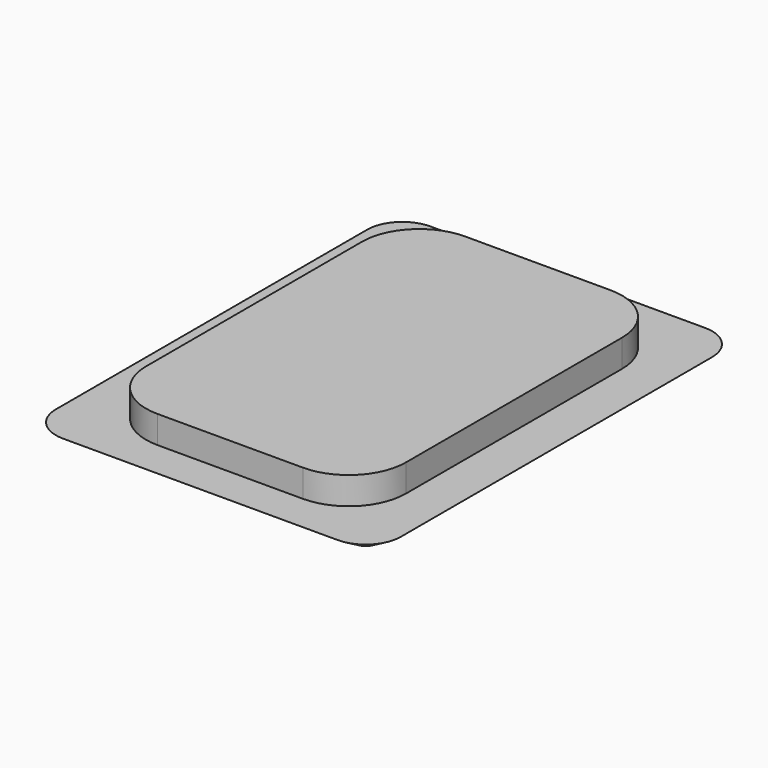
from build123d import *

# Parameters (mm, degrees)
F2_DEPTH     = 1.524
F3_DEPTH     = 0.762
F4_T1_DEPTH  = 21.59
F4_T3_DEPTH  = 15.24
F4_T6_ANGLE  = 90
F4_T8_ANGLE  = 90
F4_T10_ANGLE = 90
F4_T12_ANGLE = 90


# Not quite as in the source:
# - a fillet or chamfer that OpenCascade refuses, or shapes differently, is made with other operations: its cross-section is extruded or revolved along the edge and cut away or added


with BuildPart() as f2:
    # F1 (on face) → F2 (new body)
    with BuildSketch(Plane.XY):
        with BuildLine():
            ThreePointArc((-45.0744511747, 18.5649100114), (-44.144515205, 16.3198459811), (-41.8994511747, 15.3899100114))
            Line((-41.8994511747, 15.3899100114), (-33.8222511747, 15.3899100114))
            ThreePointArc((-33.8222511747, 15.3899100114), (-31.5771871445, 16.3198459811), (-30.6472511747, 18.5649100114))
            Line((-30.6472511747, 18.5649100114), (-30.6472511747, 33.5509100114))
            ThreePointArc((-30.6472511747, 33.5509100114), (-31.5771871445, 35.7959740417), (-33.8222511747, 36.7259100114))
            Line((-33.8222511747, 36.7259100114), (-41.8994511747, 36.7259100114))
            ThreePointArc((-41.8994511747, 36.7259100114), (-44.144515205, 35.7959740417), (-45.0744511747, 33.5509100114))
            Line((-45.0744511747, 33.5509100114), (-45.0744511747, 18.5649100114))
        make_face()
    extrude(amount=F2_DEPTH)

    # F0 (on Top) → F3 (join)
    with BuildSketch(Plane.XY):
        with BuildLine():
            ThreePointArc((-48.6558511747, 15.2629100114), (-47.725915205, 13.0178459811), (-45.4808511747, 12.0879100114))
            Line((-45.4808511747, 12.0879100114), (-30.2408511747, 12.0879100114))
            ThreePointArc((-30.2408511747, 12.0879100114), (-27.9957871445, 13.0178459811), (-27.0658511747, 15.2629100114))
            Line((-27.0658511747, 15.2629100114), (-27.0658511747, 36.8529100114))
            ThreePointArc((-27.0658511747, 36.8529100114), (-27.9957871445, 39.0979740417), (-30.2408511747, 40.0279100114))
            Line((-30.2408511747, 40.0279100114), (-45.4808511747, 40.0279100114))
            ThreePointArc((-45.4808511747, 40.0279100114), (-47.725915205, 39.0979740417), (-48.6558511747, 36.8529100114))
            Line((-48.6558511747, 36.8529100114), (-48.6558511747, 15.2629100114))
        make_face()
    extrude(amount=-F3_DEPTH)

    # F4: chamfer of 2.54 x 1.4664696837 on 8 edges, made by hand

    # F4_s2 → F4_t1 (cut)
    with BuildSketch(Plane.XZ.offset(-36.8529100114)):
        Polygon((-48.6558511747, 0.7044696837), (-46.1158511747, -0.762), (-48.6558511747, -0.762), align=None)
        Polygon((-29.6058511747, -0.762), (-27.0658511747, 0.7044696837), (-27.0658511747, -0.762), align=None)
    extrude(amount=F4_T1_DEPTH, mode=Mode.SUBTRACT)

    # F4_s4 → F4_t3 (cut)
    with BuildSketch(Plane.YZ.offset(-45.4808511747)):
        Polygon((37.4879100114, -0.762), (40.0279100114, 0.7044696837), (40.0279100114, -0.762), align=None)
        Polygon((12.0879100114, 0.7044696837), (14.6279100114, -0.762), (12.0879100114, -0.762), align=None)
    extrude(amount=F4_T3_DEPTH, mode=Mode.SUBTRACT)

    # F4_s5 → F4_t6 (revolve, cut)
    with BuildSketch(Plane.YZ.offset(-45.4808511747)):
        Polygon((37.4879100114, -0.762), (40.0279100114, 0.7044696837), (40.0279100114, -0.762), align=None)
    revolve(axis=Axis((-45.4808511747, 36.8529100114, -0.762), (0, 0, 1)), revolution_arc=F4_T6_ANGLE, mode=Mode.SUBTRACT)

    # F4_s7 → F4_t8 (revolve, cut)
    with BuildSketch(Plane.XZ.offset(-36.8529100114)):
        Polygon((-29.6058511747, -0.762), (-27.0658511747, 0.7044696837), (-27.0658511747, -0.762), align=None)
    revolve(axis=Axis((-30.2408511747, 36.8529100114, -0.762), (0, 0, 1)), revolution_arc=F4_T8_ANGLE, mode=Mode.SUBTRACT)

    # F4_s9 → F4_t10 (revolve, cut)
    with BuildSketch(Plane.YZ.offset(-30.2408511747)):
        Polygon((14.6279100114, -0.762), (12.0879100114, 0.7044696837), (12.0879100114, -0.762), align=None)
    revolve(axis=Axis((-30.2408511747, 15.2629100114, -0.762), (0, 0, 1)), revolution_arc=F4_T10_ANGLE, mode=Mode.SUBTRACT)

    # F4_s11 → F4_t12 (revolve, cut)
    with BuildSketch(Plane.XZ.offset(-15.2629100114)):
        Polygon((-48.6558511747, 0.7044696837), (-46.1158511747, -0.762), (-48.6558511747, -0.762), align=None)
    revolve(axis=Axis((-45.4808511747, 15.2629100114, -0.762), (0, 0, 1)), revolution_arc=F4_T12_ANGLE, mode=Mode.SUBTRACT)


solid = f2.part
